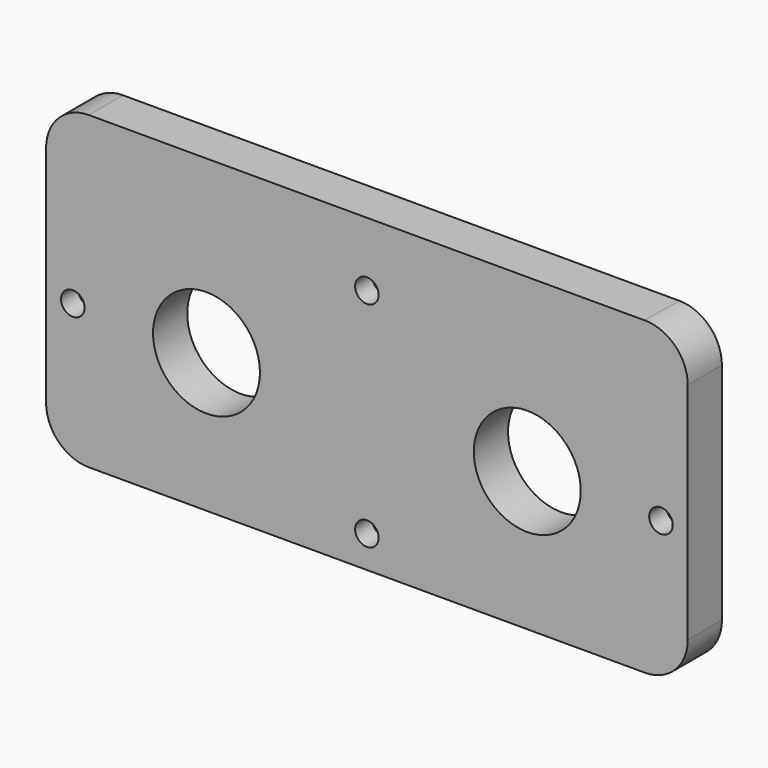
from build123d import *

# Parameters (mm, degrees)
F0_W     = 300
F0_H     = 160
F1_DEPTH = 10
F2_R     = 25
F3_DEPTH = 20.001
F4_R     = 5.5
F5_DEPTH = 10
F6_W     = 300
F6_H     = 15
F7_DEPTH = 20.001
F8_R     = 20


with BuildPart() as f1:
    # F0 (on Front) → F1 (new body, symmetric)
    with BuildSketch(Plane.XZ):
        Rectangle(F0_W, F0_H)
    extrude(amount=F1_DEPTH, both=True)

    # F2 (on face) → F3 (cut, through all)
    with BuildSketch(Plane.XZ.offset(10)):
        with Locations((-75, 0)):
            Circle(F2_R)
        with Locations((75, 0)):
            Circle(F2_R)
    extrude(amount=-F3_DEPTH, mode=Mode.SUBTRACT)

    # F4 (on face) → F5 (cut)
    with BuildSketch(Plane.XZ.offset(10)):
        with Locations((-137.5, 0)):
            Circle(F4_R)
        with Locations((0, 50)):
            Circle(F4_R)
        with Locations((137.5, 0)):
            Circle(F4_R)
        with Locations((0, -50)):
            Circle(F4_R)
    extrude(amount=-F5_DEPTH, mode=Mode.SUBTRACT)

    # F6 (on face) → F7 (cut, through all)
    with BuildSketch(Plane.XZ.offset(10)):
        with Locations((0, -72.5)):
            Rectangle(F6_W, F6_H)
    extrude(amount=-F7_DEPTH, mode=Mode.SUBTRACT)

    # F8
    f8_edges = [f1.edges().sort_by_distance(p)[0] for p in [
        (-150, 0, 80),
        (150, 0, 80),
        (-150, 0, -65),
        (150, 0, -65),
    ]]
    fillet(f8_edges, radius=F8_R)


solid = f1.part
